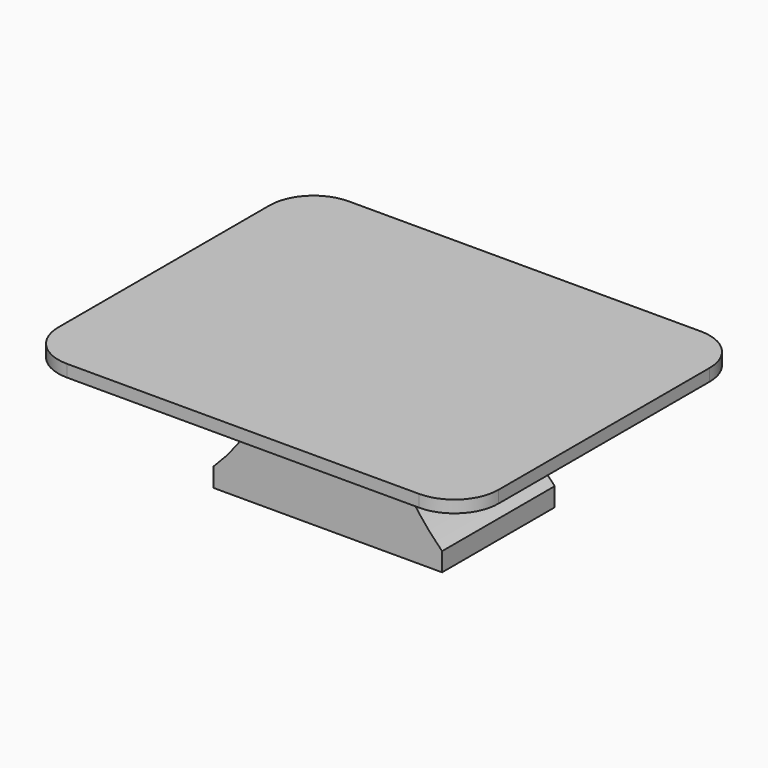
from build123d import *

# Parameters (mm, degrees)
F1_DEPTH     = 20
F2_DEPTH     = 13
F0_W         = 13
F0_H         = 2.1210866805
F3_R         = 5
F4_R         = 5
F6_DEPTH     = 8
F7_R         = 5
F8_T1_DEPTH  = 12
F8_T3_DEPTH  = 16
F8_T6_ANGLE  = 90
F8_T8_ANGLE  = 90
F8_T10_ANGLE = 90
F8_T12_ANGLE = 90


# Not quite as in the source:
# - a fillet or chamfer that OpenCascade refuses, or shapes differently, is made with other operations: its cross-section is extruded or revolved along the edge and cut away or added


with BuildPart() as f1:
    # F0 (on Front) → F1 (new body, symmetric)
    with BuildSketch(Plane.XZ):
        Polygon((0, 13.6210866805), (0, 15), (-25, 15), (-25, 13.6210866805), (-11, 13.6210866805), align=None)
        Polygon((25, 15), (0, 15), (0, 13.6210866805), (11, 13.6210866805), (25, 13.6210866805), align=None)
    extrude(amount=F1_DEPTH, both=True)

    # F0 (on Front) → F2 (join, symmetric)
    with BuildSketch(Plane.XZ):
        Polygon((0, 12.1210866805), (0, 13.6210866805), (-11, 13.6210866805), (-11, 12.1210866805), (-6.4361323602, 12.1210866805), align=None)
        Polygon((11, 13.6210866805), (0, 13.6210866805), (0, 12.1210866805), (6.4361323602, 12.1210866805), (11, 12.1210866805), align=None)
    extrude(amount=F2_DEPTH, both=True)

    # F4
    f4_edges = [f1.edges().sort_by_distance(p)[0] for p in [
        (-25, -20, 14.310543),
        (-25, 20, 14.310543),
        (25, -20, 14.310543),
        (25, 20, 14.310543),
    ]]
    fillet(f4_edges, radius=F4_R)

    # F0 (on Front) → F6 (join, symmetric)
    with BuildSketch(Plane.XZ):
        with BuildLine():
            Line((0, 2.1210866805), (0, 12.1210866805))
            Line((0, 12.1210866805), (-6.4361323602, 12.1210866805))
            ThreePointArc((-6.4361323602, 12.1210866805), (-9.1727786789, 6.7631671822), (-13, 2.1210866805))
            Line((-13, 2.1210866805), (0, 2.1210866805))
        make_face()
        with Locations((-6.5, 1.0605433403)):
            Rectangle(F0_W, F0_H)
        with BuildLine():
            Line((6.4361323602, 12.1210866805), (0, 12.1210866805))
            Line((0, 12.1210866805), (0, 2.1210866805))
            Line((0, 2.1210866805), (13, 2.1210866805))
            ThreePointArc((13, 2.1210866805), (9.1727786789, 6.7631671822), (6.4361323602, 12.1210866805))
        make_face()
        with Locations((6.5, 1.0605433403)):
            Rectangle(F0_W, F0_H)
    extrude(amount=F6_DEPTH, both=True)

    # F7
    f7_edges = [f1.edges().sort_by_distance(p)[0] for p in [
        (-11, -13, 12.871087),
        (-11, 13, 12.871087),
        (11, -13, 12.871087),
        (11, 13, 12.871087),
    ]]
    fillet(f7_edges, radius=F7_R)

    # F8: fillet of radius 5 on 1 edges, made by hand

    # F8_s2 → F8_t1 (cut)
    with BuildSketch(Plane.YZ.offset(-6)):
        with BuildLine():
            ThreePointArc((-13, 13.6210866805), (-11.3657774588, 12.5113144519), (-9.4292857857, 12.1210866805))
            Line((-9.4292857857, 12.1210866805), (-9.4292857857, 12.0210866805))
            Line((-9.4292857857, 12.0210866805), (-13, 12.0210866805))
            Line((-13, 12.0210866805), (-13.1, 12.1210866805))
            ThreePointArc((-13.1, 12.1210866805), (-13.1, 12.8710866805), (-13.0714142843, 13.5510866805))
            Line((-13.0714142843, 13.5510866805), (-13, 13.6210866805))
        make_face()
        with BuildLine():
            ThreePointArc((13, 13.6210866805), (11.3657774588, 12.5113144519), (9.4292857857, 12.1210866805))
            Line((9.4292857857, 12.1210866805), (9.4292857857, 12.0210866805))
            Line((9.4292857857, 12.0210866805), (13, 12.0210866805))
            Line((13, 12.0210866805), (13.1, 12.1210866805))
            ThreePointArc((13.1, 12.1210866805), (13.1, 12.8710866805), (13.0714142843, 13.5510866805))
            Line((13.0714142843, 13.5510866805), (13, 13.6210866805))
        make_face()
    extrude(amount=F8_T1_DEPTH, mode=Mode.SUBTRACT)

    # F8_s4 → F8_t3 (cut)
    with BuildSketch(Plane.XZ.offset(-8)):
        with BuildLine():
            ThreePointArc((11, 13.6210866805), (9.3657774588, 12.5113144519), (7.4292857857, 12.1210866805))
            Line((7.4292857857, 12.1210866805), (7.4292857857, 12.0210866805))
            Line((7.4292857857, 12.0210866805), (11, 12.0210866805))
            Line((11, 12.0210866805), (11.1, 12.1210866805))
            ThreePointArc((11.1, 12.1210866805), (11.1, 12.8710866805), (11.0714142843, 13.5510866805))
            Line((11.0714142843, 13.5510866805), (11, 13.6210866805))
        make_face()
        with BuildLine():
            ThreePointArc((-11, 13.6210866805), (-9.3657774588, 12.5113144519), (-7.4292857857, 12.1210866805))
            Line((-7.4292857857, 12.1210866805), (-7.4292857857, 12.0210866805))
            Line((-7.4292857857, 12.0210866805), (-11, 12.0210866805))
            Line((-11, 12.0210866805), (-11.1, 12.1210866805))
            ThreePointArc((-11.1, 12.1210866805), (-11.1, 12.8710866805), (-11.0714142843, 13.5510866805))
            Line((-11.0714142843, 13.5510866805), (-11, 13.6210866805))
        make_face()
    extrude(amount=F8_T3_DEPTH, mode=Mode.SUBTRACT)

    # F8_s5 → F8_t6 (revolve, cut)
    with BuildSketch(Plane.XZ.offset(8)):
        with BuildLine():
            ThreePointArc((-11, 13.6210866805), (-9.3657774588, 12.5113144519), (-7.4292857857, 12.1210866805))
            Line((-7.4292857857, 12.1210866805), (-7.4292857857, 12.0210866805))
            Line((-7.4292857857, 12.0210866805), (-11, 12.0210866805))
            Line((-11, 12.0210866805), (-11.1, 12.1210866805))
            ThreePointArc((-11.1, 12.1210866805), (-11.1, 12.8710866805), (-11.0714142843, 13.5510866805))
            Line((-11.0714142843, 13.5510866805), (-11, 13.6210866805))
        make_face()
    revolve(axis=Axis((-6, -8, 12.1210866805), (0, 0, 1)), revolution_arc=F8_T6_ANGLE, mode=Mode.SUBTRACT)

    # F8_s7 → F8_t8 (revolve, cut)
    with BuildSketch(Plane.XZ.offset(8)):
        with BuildLine():
            ThreePointArc((11, 13.6210866805), (9.3657774588, 12.5113144519), (7.4292857857, 12.1210866805))
            Line((7.4292857857, 12.1210866805), (7.4292857857, 12.0210866805))
            Line((7.4292857857, 12.0210866805), (11, 12.0210866805))
            Line((11, 12.0210866805), (11.1, 12.1210866805))
            ThreePointArc((11.1, 12.1210866805), (11.1, 12.8710866805), (11.0714142843, 13.5510866805))
            Line((11.0714142843, 13.5510866805), (11, 13.6210866805))
        make_face()
    revolve(axis=Axis((6, -8, 12.1210866805), (0, 0, -1)), revolution_arc=F8_T8_ANGLE, mode=Mode.SUBTRACT)

    # F8_s9 → F8_t10 (revolve, cut)
    with BuildSketch(Plane.YZ.offset(6)):
        with BuildLine():
            ThreePointArc((13, 13.6210866805), (11.3657774588, 12.5113144519), (9.4292857857, 12.1210866805))
            Line((9.4292857857, 12.1210866805), (9.4292857857, 12.0210866805))
            Line((9.4292857857, 12.0210866805), (13, 12.0210866805))
            Line((13, 12.0210866805), (13.1, 12.1210866805))
            ThreePointArc((13.1, 12.1210866805), (13.1, 12.8710866805), (13.0714142843, 13.5510866805))
            Line((13.0714142843, 13.5510866805), (13, 13.6210866805))
        make_face()
    revolve(axis=Axis((6, 8, 12.1210866805), (0, 0, -1)), revolution_arc=F8_T10_ANGLE, mode=Mode.SUBTRACT)

    # F8_s11 → F8_t12 (revolve, cut)
    with BuildSketch(Plane.XZ.offset(-8)):
        with BuildLine():
            ThreePointArc((-11, 13.6210866805), (-9.3657774588, 12.5113144519), (-7.4292857857, 12.1210866805))
            Line((-7.4292857857, 12.1210866805), (-7.4292857857, 12.0210866805))
            Line((-7.4292857857, 12.0210866805), (-11, 12.0210866805))
            Line((-11, 12.0210866805), (-11.1, 12.1210866805))
            ThreePointArc((-11.1, 12.1210866805), (-11.1, 12.8710866805), (-11.0714142843, 13.5510866805))
            Line((-11.0714142843, 13.5510866805), (-11, 13.6210866805))
        make_face()
    revolve(axis=Axis((-6, 8, 12.1210866805), (0, 0, -1)), revolution_arc=F8_T12_ANGLE, mode=Mode.SUBTRACT)


with BuildPart() as f2:
    # F0 (on Front) → F2, piece 2 (new body, symmetric)
    with BuildSketch(Plane.XZ):
        with Locations((-6.5, 1.0605433403)):
            Rectangle(F0_W, F0_H)
        with Locations((6.5, 1.0605433403)):
            Rectangle(F0_W, F0_H)
    extrude(amount=F2_DEPTH, both=True)

    # F3
    f3_edges = [f2.edges().sort_by_distance(p)[0] for p in [
        (-13, 13, 1.060543),
        (-13, -13, 1.060543),
        (13, -13, 1.060543),
        (13, 13, 1.060543),
    ]]
    fillet(f3_edges, radius=F3_R)


solid = f1.part
